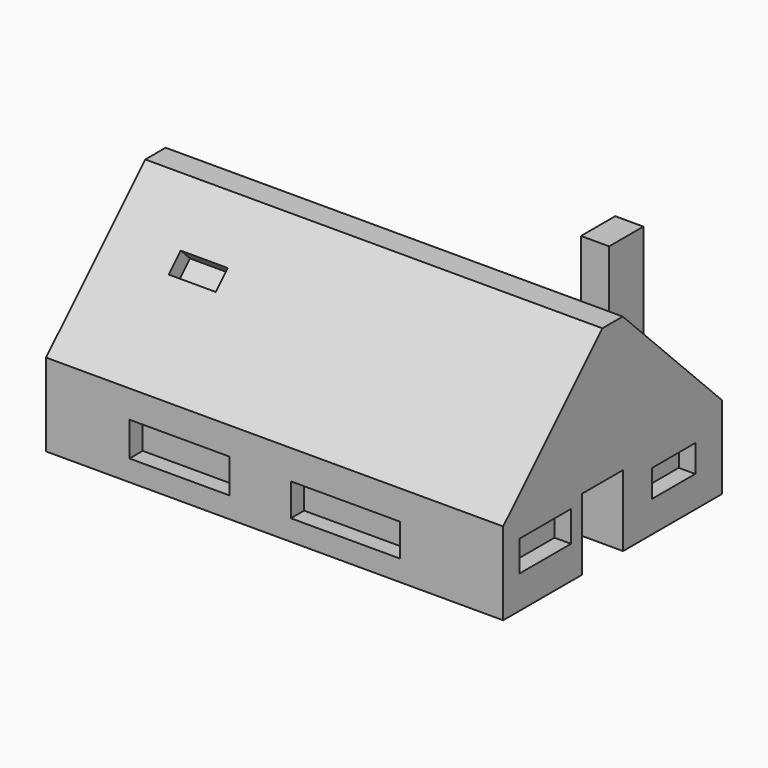
from build123d import *

# Parameters (mm, degrees)
F0_W      = 140.4484510422
F0_H      = 84.0201452374
F1_DEPTH  = 63.5
F2_SIZE   = 38.1
F3_W      = 8.6570605636
F3_H      = 13.1569579244
F4_DEPTH  = 76.2
F6_W      = 15.7950655557
F6_H      = 21.9281148165
F7_DEPTH  = 12.7
F11_W     = 16.7103528511
F11_H     = 8.3694644272
F12_DEPTH = 5.08
F13_W     = 19.7787024081
F13_H     = 9.4418320805
F14_DEPTH = 5.08
F15_W     = 30.6456126273
F15_H     = 10.5041540228
F16_DEPTH = 5.08
F17_W     = 33.5607007146
F17_H     = 9.9876374006
F18_DEPTH = 5.08
F19_W     = 21.3066544384
F19_H     = 9.7970152274
F20_DEPTH = 5.08
F21_W     = 19.7049863636
F21_H     = 9.7357481718
F22_DEPTH = 5.08
F23_W     = 27.2831916809
F23_H     = 8.0071371049
F24_DEPTH = 5.08
F25_W     = 37.1795129031
F25_H     = 7.4951220304
F26_DEPTH = 5.08
F27_W     = 14.4418329
F27_H     = 6.516110152
F28_DEPTH = 5.08
F29_W     = 17.3427406698
F29_H     = 8.6352974176
F30_DEPTH = 5.08


# Not quite as in the source:
# - the program builds the solid bodies; features that only make, move or delete a surface that nothing else refers to are left out


with BuildPart() as f1:
    # F0 (on Top) → F1 (new body)
    with BuildSketch(Plane.XY):
        with Locations((70.2242255211, -11.3064013422)):
            Rectangle(F0_W, F0_H)
    extrude(amount=F1_DEPTH)

    # F2
    f2_edges = [f1.edges().sort_by_distance(p)[0] for p in [
        (70.224226, -53.316474, 63.5),
        (70.224226, 30.703671, 63.5),
    ]]
    chamfer(f2_edges, length=F2_SIZE)

    # F6 (on face) → F7 (cut)
    with BuildSketch(Plane.YZ.offset(140.4484510422)):
        with Locations((-15.1667564642, 10.9640574083)):
            Rectangle(F6_W, F6_H)
    extrude(amount=-F7_DEPTH, mode=Mode.SUBTRACT)

    # F11 (on face) → F12 (cut)
    with BuildSketch(Plane.YZ.offset(140.4484510422)):
        with Locations((12.1226046467, 13.7810688466)):
            Rectangle(F11_W, F11_H)
    extrude(amount=-F12_DEPTH, mode=Mode.SUBTRACT)

    # F13 (on face) → F14 (cut)
    with BuildSketch(Plane.YZ.offset(140.4484510422)):
        with Locations((-37.1385682374, 14.8160951212)):
            Rectangle(F13_W, F13_H)
    extrude(amount=-F14_DEPTH, mode=Mode.SUBTRACT)

    # F15 (on face) → F16 (cut)
    with BuildSketch(Plane.XZ.offset(53.3164739609)):
        with Locations((40.9622769803, 11.6851397324)):
            Rectangle(F15_W, F15_H)
    extrude(amount=-F16_DEPTH, mode=Mode.SUBTRACT)

    # F17 (on face) → F18 (cut)
    with BuildSketch(Plane.XZ.offset(53.3164739609)):
        with Locations((91.9907130301, 11.3846212626)):
            Rectangle(F17_W, F17_H)
    extrude(amount=-F18_DEPTH, mode=Mode.SUBTRACT)

    # F19 (on face) → F20 (cut)
    with BuildSketch(Plane(origin=(0, 0, 0), x_dir=(0, -1, 0), z_dir=(-1, 0, 0))):
        with Locations((-10.6533272192, 14.9779669009)):
            Rectangle(F19_W, F19_H)
    extrude(amount=-F20_DEPTH, mode=Mode.SUBTRACT)

    # F21 (on face) → F22 (cut)
    with BuildSketch(Plane(origin=(0, 0, 0), x_dir=(0, -1, 0), z_dir=(-1, 0, 0))):
        with Locations((24.8714331537, 14.5110972226)):
            Rectangle(F21_W, F21_H)
    extrude(amount=-F22_DEPTH, mode=Mode.SUBTRACT)

    # F23 (on face) → F24 (cut)
    with BuildSketch(Plane(origin=(0, 30.7036712766, 0), x_dir=(-1, 0, 0), z_dir=(0, 1, 0))):
        with Locations((-108.3185896277, 12.4019039795)):
            Rectangle(F23_W, F23_H)
    extrude(amount=-F24_DEPTH, mode=Mode.SUBTRACT)

    # F25 (on face) → F26 (cut)
    with BuildSketch(Plane(origin=(0, 30.7036712766, 0), x_dir=(-1, 0, 0), z_dir=(0, 1, 0))):
        with Locations((-46.9700554386, 11.6554377601)):
            Rectangle(F25_W, F25_H)
    extrude(amount=-F26_DEPTH, mode=Mode.SUBTRACT)

    # F27 (on face) → F28 (cut)
    with BuildSketch(Plane(origin=(0, -39.3582369804, 39.3582369804), x_dir=(1, 0, 0), z_dir=(0, -0.7071067812, 0.7071067812))):
        with Locations((28.2577574253, 12.9630696028)):
            Rectangle(F27_W, F27_H)
    extrude(amount=-F28_DEPTH, mode=Mode.SUBTRACT)

    # F29 (on face) → F30 (cut)
    with BuildSketch(Plane(origin=(0, 28.0518356383, 28.0518356383), x_dir=(-1, 0, 0), z_dir=(0, 0.7071067812, 0.7071067812))):
        with Locations((-26.6702575609, 27.6306420565)):
            Rectangle(F29_W, F29_H)
    extrude(amount=-F30_DEPTH, mode=Mode.SUBTRACT)


with BuildPart() as f4:
    # F3 (on Top) → F4 (new body)
    with BuildSketch(Plane.XY):
        with Locations((126.0326392949, 6.5784789622)):
            Rectangle(F3_W, F3_H)
    extrude(amount=F4_DEPTH)


solid = Compound([f1.part, f4.part])
